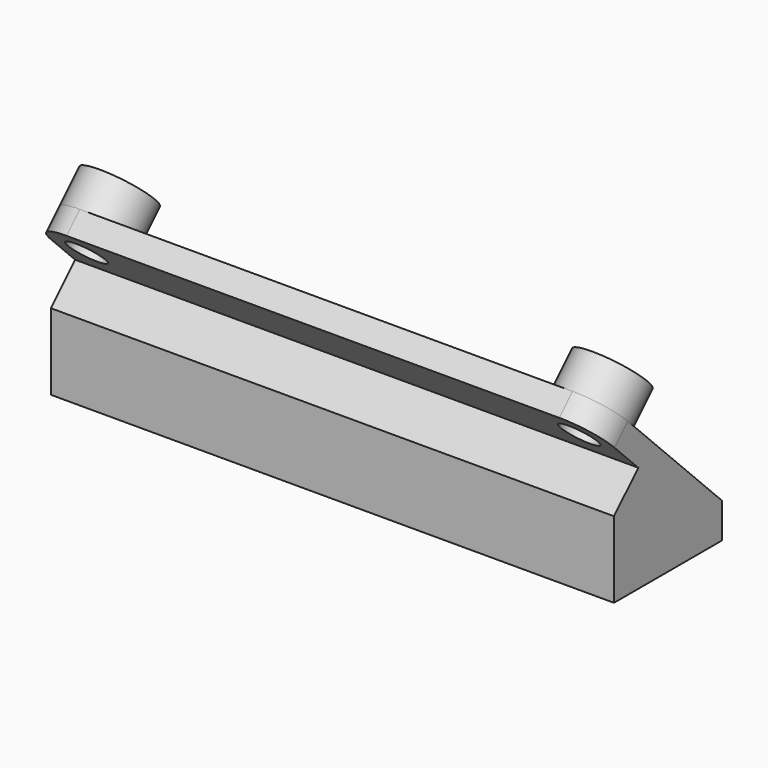
from build123d import *

# Parameters (mm, degrees)
F0_W          = 48
F0_H          = 11.5
F1_DEPTH      = 20
F2_W          = 46
F2_H          = 9.5
F3_DEPTH      = 3
F5_DEPTH      = 40
F5_DEPTH_BACK = 40
F7_D          = 5
F7_DEPTH      = 10
F7_START      = 2
F7_TIP        = 1.5021515476
F9_W          = 48
F9_H          = 9.6
F10_DEPTH     = 2
F11_R         = 3
F12_DEPTH     = 3
F13_R         = 1.6
F14_DEPTH     = 12.5
F15_R         = 2.9999


# Not quite as in the source:
# - a fillet or chamfer is up to 0.001 mm smaller than in the source, because OpenCascade refuses the exact size
# - a feature names something its author has since deleted; it is built from what else it names


with BuildPart() as f1:
    # F0 (on Top) → F1 (new body)
    with BuildSketch(Plane.XY):
        with Locations((4.8962971196, -3.7300640109)):
            Rectangle(F0_W, F0_H)
    extrude(amount=F1_DEPTH)

    # F2 (on Top) → F3 (cut)
    with BuildSketch(Plane.XY):
        with Locations((4.8962971196, -3.7300640109)):
            Rectangle(F2_W, F2_H)
    extrude(amount=F3_DEPTH, mode=Mode.SUBTRACT)

    # F4 (on Right) → F5 (cut, two sides)
    with BuildSketch(Plane.YZ) as f5_sk:
        Polygon((-5.4800640109, 10.5), (2.0199359891, 3), (2.0199359891, 33), (-12.9800640109, 33), (-12.9800640109, 3), align=None)
    extrude(amount=F5_DEPTH, mode=Mode.SUBTRACT)
    extrude(f5_sk.sketch, amount=-F5_DEPTH_BACK, mode=Mode.SUBTRACT)

    # F7
    # its depths count from where the whole tool has entered the part; down to there all is cleared
    with Locations(Plane(origin=(0, 2.5099679945, 2.5099679945), x_dir=(-1, 0, 0), z_dir=(0, 0.7071067812, 0.7071067812)).offset(-F7_START)):
        with Locations((-10.3962971196, 1.1930099081)):
            Hole(F7_D / 2, depth=F7_DEPTH)
            with Locations((0, 0, -(F7_DEPTH + F7_TIP / 2))):  # 118° drill point
                Cone(0, F7_D / 2, F7_TIP, mode=Mode.SUBTRACT)

    # F9 (on offset) → F10 (join)
    with BuildSketch(Plane(origin=(0, 2.5099679945, 2.5099679945), x_dir=(-1, 0, 0), z_dir=(0, 0.7071067812, 0.7071067812))):
        with Locations((-4.8962971196, 13.0996116259)):
            Rectangle(F9_W, F9_H)
    extrude(amount=-F10_DEPTH)

    # F11 (on offset) → F12 (join)
    with BuildSketch(Plane(origin=(0, 2.5099679945, 2.5099679945), x_dir=(-1, 0, 0), z_dir=(0, 0.7071067812, 0.7071067812))):
        with Locations((16.1037028804, 14.8996116259)):
            Circle(F11_R)
        with Locations((-25.8962971196, 14.8996116259)):
            Circle(F11_R)
    extrude(amount=F12_DEPTH)

    # F13 (on offset) → F14 (cut, symmetric)
    with BuildSketch(Plane(origin=(0, 2.5099679945, 2.5099679945), x_dir=(-1, 0, 0), z_dir=(0, 0.7071067812, 0.7071067812))):
        with Locations((16.1037028804, 14.8996116259)):
            Circle(F13_R)
        with Locations((-25.8962971196, 14.8996116259)):
            Circle(F13_R)
    extrude(amount=F14_DEPTH, both=True, mode=Mode.SUBTRACT)

    # F15 (radius 3 in the source; OpenCascade refuses exactly that, so slightly less here)
    f15_edges = [f1.edges().sort_by_distance(p)[0] for p in [
        (-19.103703, -10.854076, 14.459798),
        (28.896297, -10.854076, 14.459798),
    ]]
    fillet(f15_edges, radius=F15_R)


solid = f1.part
